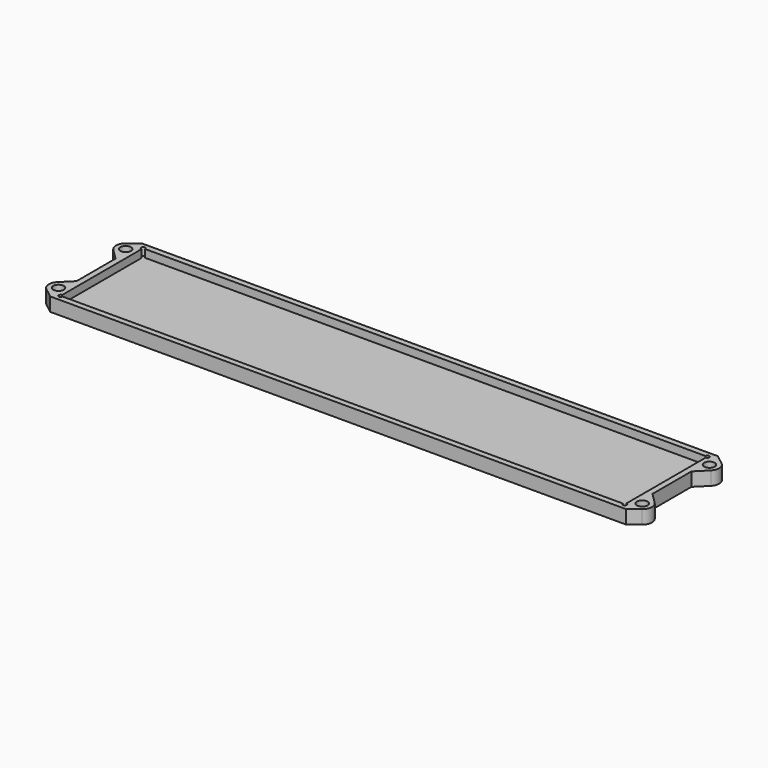
from build123d import *

# Parameters (mm, degrees)
F0_W     = 234.762548
F0_H     = 46.762416
F0_W_2   = 230.000048
F0_H_2   = 41.999916
F1_DEPTH = 3.175
F2_W     = 234.762548
F2_H     = 46.762416
F3_DEPTH = 2.38125
F5_DEPTH = 5.55625
F6_R     = 2.15265
F7_DEPTH = 5.55625
F8_R     = 0.79375
F9_DEPTH = 3.175


# Not quite as in the source:
# - a length typed as a fraction of an inch, garbled in the dataset ("3 / 203.2 mm" for 3/8 in), is restored


with BuildPart() as f1:
    # F0 (on Top) → F1 (new body)
    with BuildSketch(Plane.XY):
        Rectangle(F0_W, F0_H)
        Rectangle(F0_W_2, F0_H_2, mode=Mode.SUBTRACT)
    extrude(amount=F1_DEPTH)

    # F2 (on face) → F3 (join)
    with BuildSketch(Plane(origin=(0, 0, 0), x_dir=(1, 0, 0), z_dir=(0, 0, -1))):
        Rectangle(F2_W, F2_H)
    extrude(amount=F3_DEPTH)

    # F4 (on face) → F5 (join, through all)
    with BuildSketch(Plane(origin=(0, 0, -2.38125), x_dir=(1, 0, 0), z_dir=(0, 0, -1))):
        with BuildLine():
            Line((-121.408854552, -20.241406366), (-117.381274, -23.381208))
            Line((-117.381274, -23.381208), (-117.381274, -9.9112329577))
            Line((-117.381274, -9.9112329577), (-121.7751040378, -14.3050629955))
            ThreePointArc((-121.7751040378, -14.3050629955), (-122.9299921425, -17.3557849119), (-121.408854552, -20.241406366))
        make_face()
        with BuildLine():
            Line((-117.381274, 9.9112329577), (-117.381274, 23.381208))
            Line((-117.381274, 23.381208), (-121.408854552, 20.241406366))
            ThreePointArc((-121.408854552, 20.241406366), (-122.9299921425, 17.3557849119), (-121.7751040378, 14.3050629955))
            Line((-121.7751040378, 14.3050629955), (-117.381274, 9.9112329577))
        make_face()
        with BuildLine():
            Line((117.381274, -9.9112329577), (117.381274, -23.381208))
            Line((117.381274, -23.381208), (121.408854552, -20.241406366))
            ThreePointArc((121.408854552, -20.241406366), (122.9299921425, -17.3557849119), (121.7751040378, -14.3050629955))
            Line((121.7751040378, -14.3050629955), (117.381274, -9.9112329577))
        make_face()
        with BuildLine():
            Line((121.408854552, 20.241406366), (117.381274, 23.381208))
            Line((117.381274, 23.381208), (117.381274, 9.9112329577))
            Line((117.381274, 9.9112329577), (121.7751040378, 14.3050629955))
            ThreePointArc((121.7751040378, 14.3050629955), (122.9299921425, 17.3557849119), (121.408854552, 20.241406366))
        make_face()
    extrude(amount=-F5_DEPTH)

    # F6 (on face) → F7 (cut, through all)
    with BuildSketch(Plane(origin=(0, 0, -2.38125), x_dir=(1, 0, 0), z_dir=(0, 0, -1))):
        with Locations((-118.968774, -17.1113930333)):
            Circle(F6_R)
        with Locations((-118.968774, 17.1113930333)):
            Circle(F6_R)
        with Locations((118.968774, 17.1113930333)):
            Circle(F6_R)
        with Locations((118.968774, -17.1113930333)):
            Circle(F6_R)
    extrude(amount=-F7_DEPTH, mode=Mode.SUBTRACT)

    # F8 (on face) → F9 (cut, through all)
    with BuildSketch(Plane.XY.offset(3.175)):
        with Locations((-115.000024, 20.999958)):
            Circle(F8_R)
        with Locations((-115.000024, -20.999958)):
            Circle(F8_R)
        with Locations((115.000024, -20.999958)):
            Circle(F8_R)
        with Locations((115.000024, 20.999958)):
            Circle(F8_R)
    extrude(amount=-F9_DEPTH, mode=Mode.SUBTRACT)


solid = f1.part
